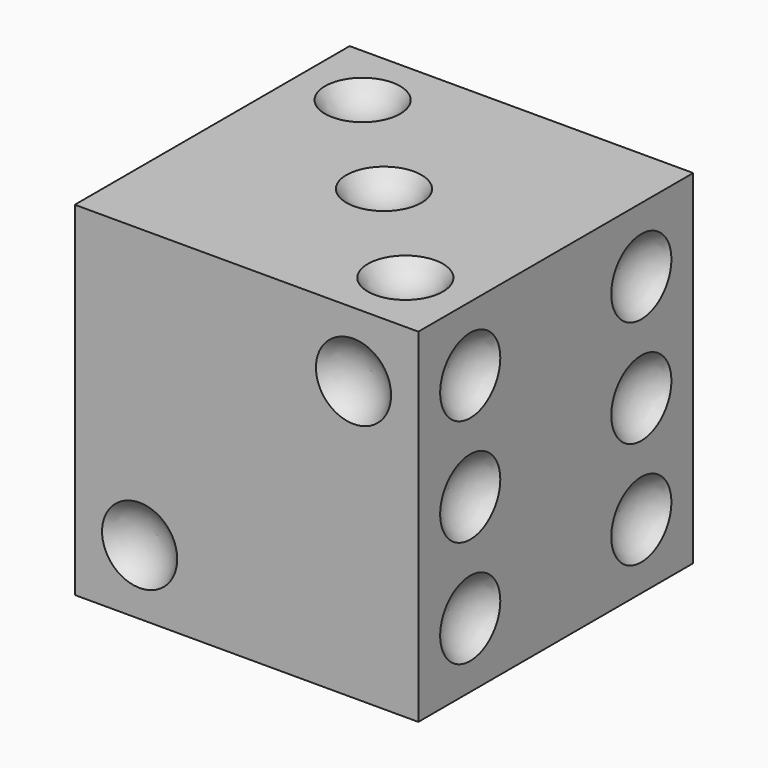
from build123d import *

# Parameters (mm, degrees)
F0_W      = 16
F0_H      = 16
F1_DEPTH  = 8
F2_R      = 1.75
F3_DEPTH  = 1
F4_R      = 1.75
F5_DEPTH  = 1
F6_R      = 1.75
F7_DEPTH  = 1
F8_R      = 1.75
F9_DEPTH  = 1
F10_R     = 1.75
F11_DEPTH = 1
F12_R     = 1.75
F13_DEPTH = 1


# Not quite as in the source:
# - a fillet or chamfer that OpenCascade refuses, or shapes differently, is made with other operations: its cross-section is extruded or revolved along the edge and cut away or added


with BuildPart() as f1:
    # F0 (on Top) → F1 (new body, symmetric)
    with BuildSketch(Plane.XY):
        Rectangle(F0_W, F0_H)
    extrude(amount=F1_DEPTH, both=True)

    # F2 (on face) → F3 (cut)
    with BuildSketch(Plane.XY.offset(8)):
        Circle(F2_R)
        with Locations((-4.98, 4.98)):
            Circle(F2_R)
        with Locations((4.98, -4.98)):
            Circle(F2_R)
    extrude(amount=-F3_DEPTH, mode=Mode.SUBTRACT)

    # F4 (on face) → F5 (cut)
    with BuildSketch(Plane.XZ.offset(8)):
        with Locations((4.98, 4.98)):
            Circle(F4_R)
        with Locations((-4.98, -4.98)):
            Circle(F4_R)
    extrude(amount=-F5_DEPTH, mode=Mode.SUBTRACT)

    # F6 (on face) → F7 (cut)
    with BuildSketch(Plane(origin=(-8, 0, 0), x_dir=(0, -1, 0), z_dir=(-1, 0, 0))):
        Circle(F6_R)
    extrude(amount=-F7_DEPTH, mode=Mode.SUBTRACT)

    # F8 (on face) → F9 (cut)
    with BuildSketch(Plane(origin=(0, 8, 0), x_dir=(-1, 0, 0), z_dir=(0, 1, 0))):
        Circle(F8_R)
        with Locations((-4.98, 4.98)):
            Circle(F8_R)
        with Locations((4.98, 4.98)):
            Circle(F8_R)
        with Locations((4.98, -4.98)):
            Circle(F8_R)
        with Locations((-4.98, -4.98)):
            Circle(F8_R)
    extrude(amount=-F9_DEPTH, mode=Mode.SUBTRACT)

    # F10 (on face) → F11 (cut)
    with BuildSketch(Plane(origin=(0, 0, -8), x_dir=(1, 0, 0), z_dir=(0, 0, -1))):
        with Locations((-4.98, 4.98)):
            Circle(F10_R)
        with Locations((4.98, 4.98)):
            Circle(F10_R)
        with Locations((4.98, -4.98)):
            Circle(F10_R)
        with Locations((-4.98, -4.98)):
            Circle(F10_R)
    extrude(amount=-F11_DEPTH, mode=Mode.SUBTRACT)

    # F12 (on face) → F13 (cut)
    with BuildSketch(Plane.YZ.offset(8)):
        with Locations((-4.98, 4.98)):
            Circle(F12_R)
        with Locations((-4.98, 0)):
            Circle(F12_R)
        with Locations((-4.98, -4.98)):
            Circle(F12_R)
        with Locations((4.98, -4.98)):
            Circle(F12_R)
        with Locations((4.98, 0)):
            Circle(F12_R)
        with Locations((4.98, 4.98)):
            Circle(F12_R)
    extrude(amount=-F13_DEPTH, mode=Mode.SUBTRACT)

    # F14: fillet of radius 2.01 on 21 edges, made by hand

    # F14_s1 → F14_t2 (revolve)
    with BuildSketch(Plane.XZ.offset(4.98)):
        with BuildLine():
            ThreePointArc((6.73, 8), (5.9946821631, 7.2678461606), (4.9921852803, 7))
            Line((4.9921852803, 7), (6.73, 7))
            Line((6.73, 7), (6.73, 8))
        make_face()
    revolve(axis=Axis((4.98, -4.98, 7), (0, 0, 1)))

    # F14_s3 → F14_t4 (revolve)
    with BuildSketch(Plane.XZ):
        with BuildLine():
            ThreePointArc((1.75, 8), (1.0146821631, 7.2678461606), (0.0121852803, 7))
            Line((0.0121852803, 7), (1.75, 7))
            Line((1.75, 7), (1.75, 8))
        make_face()
    revolve(axis=Axis((0, 0, 7), (0, 0, 1)))

    # F14_s5 → F14_t6 (revolve)
    with BuildSketch(Plane.XZ.offset(-4.98)):
        with BuildLine():
            ThreePointArc((-3.23, 8), (-3.9653178369, 7.2678461606), (-4.9678147197, 7))
            Line((-4.9678147197, 7), (-3.23, 7))
            Line((-3.23, 7), (-3.23, 8))
        make_face()
    revolve(axis=Axis((-4.98, 4.98, 7), (0, 0, 1)))

    # F14_s7 → F14_t8 (revolve)
    with BuildSketch(Plane.XY.offset(4.98)):
        with BuildLine():
            ThreePointArc((6.73, -8), (5.9946821631, -7.2678461606), (4.9921852803, -7))
            Line((4.9921852803, -7), (6.73, -7))
            Line((6.73, -7), (6.73, -8))
        make_face()
    revolve(axis=Axis((4.98, -7, 4.98), (0, -1, 0)))

    # F14_s9 → F14_t10 (revolve)
    with BuildSketch(Plane.XY.offset(-4.98)):
        with BuildLine():
            ThreePointArc((-3.23, -8), (-3.9653178369, -7.2678461606), (-4.9678147197, -7))
            Line((-4.9678147197, -7), (-3.23, -7))
            Line((-3.23, -7), (-3.23, -8))
        make_face()
    revolve(axis=Axis((-4.98, -7, -4.98), (0, -1, 0)))

    # F14_s11 → F14_t12 (revolve)
    with BuildSketch(Plane.XY):
        with BuildLine():
            ThreePointArc((-8, -1.75), (-7.2678461606, -1.0146821631), (-7, -0.0121852803))
            Line((-7, -0.0121852803), (-7, -1.75))
            Line((-7, -1.75), (-8, -1.75))
        make_face()
    revolve(axis=Axis((-7, 0, 0), (-1, 0, 0)))

    # F14_s13 → F14_t14 (revolve)
    with BuildSketch(Plane.XY.offset(4.98)):
        with BuildLine():
            ThreePointArc((3.23, 8), (3.9653178369, 7.2678461606), (4.9678147197, 7))
            Line((4.9678147197, 7), (3.23, 7))
            Line((3.23, 7), (3.23, 8))
        make_face()
    revolve(axis=Axis((4.98, 7, 4.98), (0, 1, 0)))

    # F14_s15 → F14_t16 (revolve)
    with BuildSketch(Plane.XY):
        with BuildLine():
            ThreePointArc((-1.75, 8), (-1.0146821631, 7.2678461606), (-0.0121852803, 7))
            Line((-0.0121852803, 7), (-1.75, 7))
            Line((-1.75, 7), (-1.75, 8))
        make_face()
    revolve(axis=Axis((0, 7, 0), (0, 1, 0)))

    # F14_s17 → F14_t18 (revolve)
    with BuildSketch(Plane.XY.offset(4.98)):
        with BuildLine():
            ThreePointArc((-6.73, 8), (-5.9946821631, 7.2678461606), (-4.9921852803, 7))
            Line((-4.9921852803, 7), (-6.73, 7))
            Line((-6.73, 7), (-6.73, 8))
        make_face()
    revolve(axis=Axis((-4.98, 7, 4.98), (0, 1, 0)))

    # F14_s19 → F14_t20 (revolve)
    with BuildSketch(Plane.XY.offset(-4.98)):
        with BuildLine():
            ThreePointArc((-6.73, 8), (-5.9946821631, 7.2678461606), (-4.9921852803, 7))
            Line((-4.9921852803, 7), (-6.73, 7))
            Line((-6.73, 7), (-6.73, 8))
        make_face()
    revolve(axis=Axis((-4.98, 7, -4.98), (0, 1, 0)))

    # F14_s21 → F14_t22 (revolve)
    with BuildSketch(Plane.XY.offset(-4.98)):
        with BuildLine():
            ThreePointArc((3.23, 8), (3.9653178369, 7.2678461606), (4.9678147197, 7))
            Line((4.9678147197, 7), (3.23, 7))
            Line((3.23, 7), (3.23, 8))
        make_face()
    revolve(axis=Axis((4.98, 7, -4.98), (0, 1, 0)))

    # F14_s23 → F14_t24 (revolve)
    with BuildSketch(Plane.XZ.offset(4.98)):
        with BuildLine():
            ThreePointArc((-3.23, -8), (-3.9653178369, -7.2678461606), (-4.9678147197, -7))
            Line((-4.9678147197, -7), (-3.23, -7))
            Line((-3.23, -7), (-3.23, -8))
        make_face()
    revolve(axis=Axis((-4.98, -4.98, -7), (0, 0, -1)))

    # F14_s25 → F14_t26 (revolve)
    with BuildSketch(Plane.XZ.offset(4.98)):
        with BuildLine():
            ThreePointArc((6.73, -8), (5.9946821631, -7.2678461606), (4.9921852803, -7))
            Line((4.9921852803, -7), (6.73, -7))
            Line((6.73, -7), (6.73, -8))
        make_face()
    revolve(axis=Axis((4.98, -4.98, -7), (0, 0, -1)))

    # F14_s27 → F14_t28 (revolve)
    with BuildSketch(Plane.XZ.offset(-4.98)):
        with BuildLine():
            ThreePointArc((6.73, -8), (5.9946821631, -7.2678461606), (4.9921852803, -7))
            Line((4.9921852803, -7), (6.73, -7))
            Line((6.73, -7), (6.73, -8))
        make_face()
    revolve(axis=Axis((4.98, 4.98, -7), (0, 0, -1)))

    # F14_s29 → F14_t30 (revolve)
    with BuildSketch(Plane.XZ.offset(-4.98)):
        with BuildLine():
            ThreePointArc((-3.23, -8), (-3.9653178369, -7.2678461606), (-4.9678147197, -7))
            Line((-4.9678147197, -7), (-3.23, -7))
            Line((-3.23, -7), (-3.23, -8))
        make_face()
    revolve(axis=Axis((-4.98, 4.98, -7), (0, 0, -1)))

    # F14_s31 → F14_t32 (revolve)
    with BuildSketch(Plane.XY):
        with BuildLine():
            ThreePointArc((8, 6.73), (7.2678461606, 5.9946821631), (7, 4.9921852803))
            Line((7, 4.9921852803), (7, 6.73))
            Line((7, 6.73), (8, 6.73))
        make_face()
    revolve(axis=Axis((7, 4.98, 0), (1, 0, 0)))

    # F14_s33 → F14_t34 (revolve)
    with BuildSketch(Plane.XY.offset(-4.98)):
        with BuildLine():
            ThreePointArc((8, 6.73), (7.2678461606, 5.9946821631), (7, 4.9921852803))
            Line((7, 4.9921852803), (7, 6.73))
            Line((7, 6.73), (8, 6.73))
        make_face()
    revolve(axis=Axis((7, 4.98, -4.98), (1, 0, 0)))

    # F14_s35 → F14_t36 (revolve)
    with BuildSketch(Plane.XY.offset(-4.98)):
        with BuildLine():
            ThreePointArc((8, -3.23), (7.2678461606, -3.9653178369), (7, -4.9678147197))
            Line((7, -4.9678147197), (7, -3.23))
            Line((7, -3.23), (8, -3.23))
        make_face()
    revolve(axis=Axis((7, -4.98, -4.98), (1, 0, 0)))

    # F14_s37 → F14_t38 (revolve)
    with BuildSketch(Plane.XY):
        with BuildLine():
            ThreePointArc((8, -3.23), (7.2678461606, -3.9653178369), (7, -4.9678147197))
            Line((7, -4.9678147197), (7, -3.23))
            Line((7, -3.23), (8, -3.23))
        make_face()
    revolve(axis=Axis((7, -4.98, 0), (1, 0, 0)))

    # F14_s39 → F14_t40 (revolve)
    with BuildSketch(Plane.XY.offset(4.98)):
        with BuildLine():
            ThreePointArc((8, -3.23), (7.2678461606, -3.9653178369), (7, -4.9678147197))
            Line((7, -4.9678147197), (7, -3.23))
            Line((7, -3.23), (8, -3.23))
        make_face()
    revolve(axis=Axis((7, -4.98, 4.98), (1, 0, 0)))

    # F14_s41 → F14_t42 (revolve)
    with BuildSketch(Plane.XY.offset(4.98)):
        with BuildLine():
            ThreePointArc((8, 6.73), (7.2678461606, 5.9946821631), (7, 4.9921852803))
            Line((7, 4.9921852803), (7, 6.73))
            Line((7, 6.73), (8, 6.73))
        make_face()
    revolve(axis=Axis((7, 4.98, 4.98), (1, 0, 0)))


solid = f1.part
